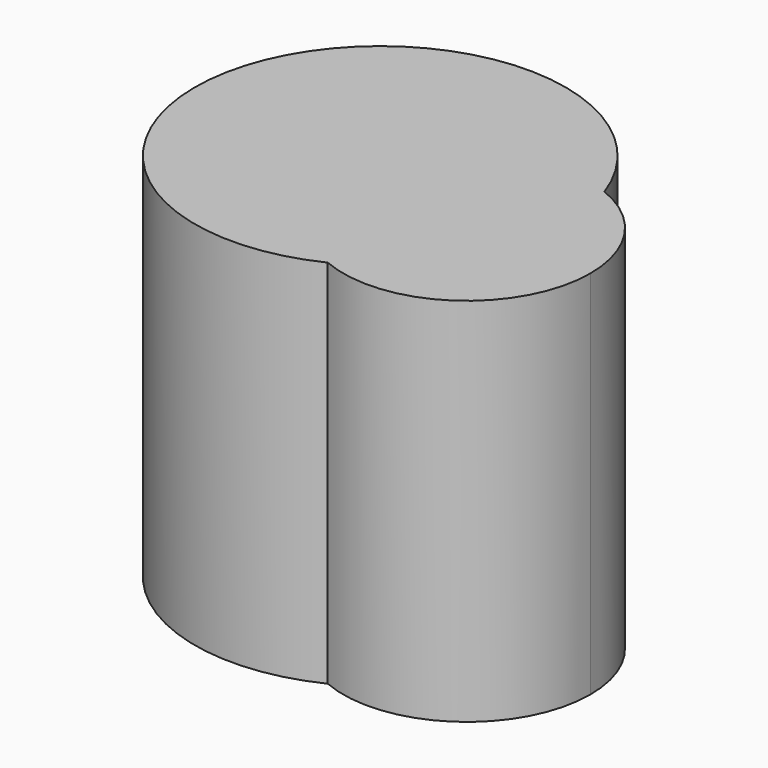
from build123d import *

# Parameters (mm, degrees)
F1_DEPTH = 76.2


# Not quite as in the source:
# - the program builds the solid bodies; features that only make, move or delete a surface that nothing else refers to are left out


with BuildPart() as f1:
    # F0 (on Top) → F1 (new body)
    with BuildSketch(Plane.XY):
        with BuildLine():
            ThreePointArc((25.4, 0), (21.0288529546, 14.2459588449), (9.4198942195, 23.5886750983))
            ThreePointArc((9.4198942195, 23.5886750983), (11.0530358989, 17.3262879854), (11.6027031443, 10.8778377828))
            ThreePointArc((11.6027031443, 10.8778377828), (5.7908709636, -9.3479927037), (-9.8715340666, -23.4032650536))
            ThreePointArc((-9.8715340666, -23.4032650536), (14.0432018199, -21.1647934704), (25.4, 0))
        make_face()
        with BuildLine():
            ThreePointArc((-27.7389652249, 48.9575995948), (-26.3638524464, 42.2521457464), (-25.9026905717, 35.4226965598))
            ThreePointArc((-25.9026905717, 35.4226965598), (-34.4786287625, 7.1778987321), (-57.3109033406, -11.530456561))
            ThreePointArc((-57.3109033406, -11.530456561), (-35.747411588, -26.0822133189), (-9.8715340666, -23.4032650536))
            ThreePointArc((-9.8715340666, -23.4032650536), (-23.4970552293, 9.6461596271), (9.4198942195, 23.5886750983))
            ThreePointArc((9.4198942195, 23.5886750983), (-5.0148958898, 42.3439536654), (-27.7389652249, 48.9575995948))
        make_face()
        with BuildLine():
            ThreePointArc((-57.3109033406, -11.530456561), (-34.4786287625, 7.1778987321), (-25.9026905717, 35.4226965598))
            ThreePointArc((-25.9026905717, 35.4226965598), (-26.3638524464, 42.2521457464), (-27.7389652249, 48.9575995948))
            ThreePointArc((-27.7389652249, 48.9575995948), (-60.7257411071, 27.6117436069), (-57.3109033406, -11.530456561))
        make_face()
        with BuildLine():
            ThreePointArc((11.6027031443, 10.8778377828), (11.0530358989, 17.3262879854), (9.4198942195, 23.5886750983))
            ThreePointArc((9.4198942195, 23.5886750983), (-23.4970552293, 9.6461596271), (-9.8715340666, -23.4032650536))
            ThreePointArc((-9.8715340666, -23.4032650536), (5.7908709636, -9.3479927037), (11.6027031443, 10.8778377828))
        make_face()
    extrude(amount=F1_DEPTH)


solid = f1.part
